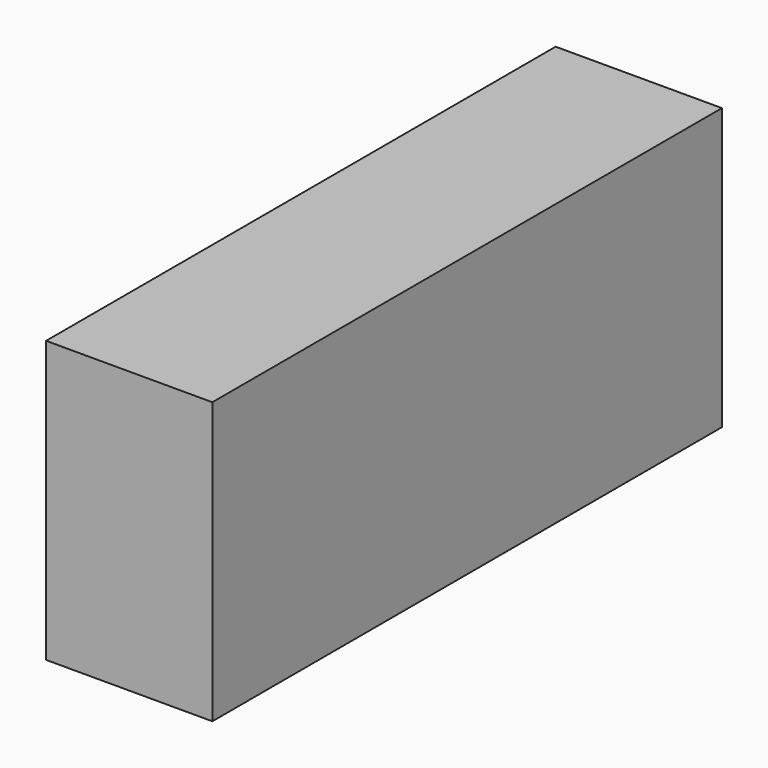
from build123d import *

# Parameters (mm, degrees)
F0_W          = 43
F0_H          = 77
F1_DEPTH      = 181
F2_W          = 50.9000002146
F2_H          = 86
F2_W_2        = 46.9000002146
F2_H_2        = 82
F3_DEPTH      = 181
F3_DEPTH_BACK = 10
F4_R          = 8
F5_W          = 50.9000002146
F5_H          = 86
F6_DEPTH      = 2
F7_W          = 50.9000002146
F7_H          = 86
F8_DEPTH      = 2


# Not quite as in the source:
# - a feature names something its author has since deleted; it is built from what else it names


with BuildPart() as f1:
    # F0 (on Front) → F1 (new body)
    with BuildSketch(Plane.XZ):
        Rectangle(F0_W, F0_H)
    extrude(amount=F1_DEPTH)


with BuildPart() as f3:
    # F2 (on face) → F3 (new body, two sides)
    with BuildSketch(Plane.XZ.offset(181)) as f3_sk:
        with Locations((-0.5499998927, 0)):
            Rectangle(F2_W, F2_H)
        with Locations((-0.5499998927, 0)):
            Rectangle(F2_W_2, F2_H_2, mode=Mode.SUBTRACT)
    extrude(amount=-F3_DEPTH)
    extrude(f3_sk.sketch, amount=F3_DEPTH_BACK)

    # F4
    f4_edges = [f3.edges().sort_by_distance(p)[0] for p in [
        (-24, -95.5, 41),
        (22.9, -95.5, 41),
        (22.9, -95.5, -41),
        (-24, -95.5, -41),
    ]]
    fillet(f4_edges, radius=F4_R)

    # F5 (on face) → F6 (join)
    with BuildSketch(Plane(origin=(0, 0, 0), x_dir=(-1, 0, 0), z_dir=(0, 1, 0))):
        with Locations((0.5499998927, 0)):
            Rectangle(F5_W, F5_H)
    extrude(amount=F6_DEPTH)

    # F7 (on face) → F8 (join)
    with BuildSketch(Plane.XZ.offset(191)):
        with Locations((-0.5499998927, 0)):
            Rectangle(F7_W, F7_H)
    extrude(amount=F8_DEPTH)


solid = Compound([f1.part, f3.part])
